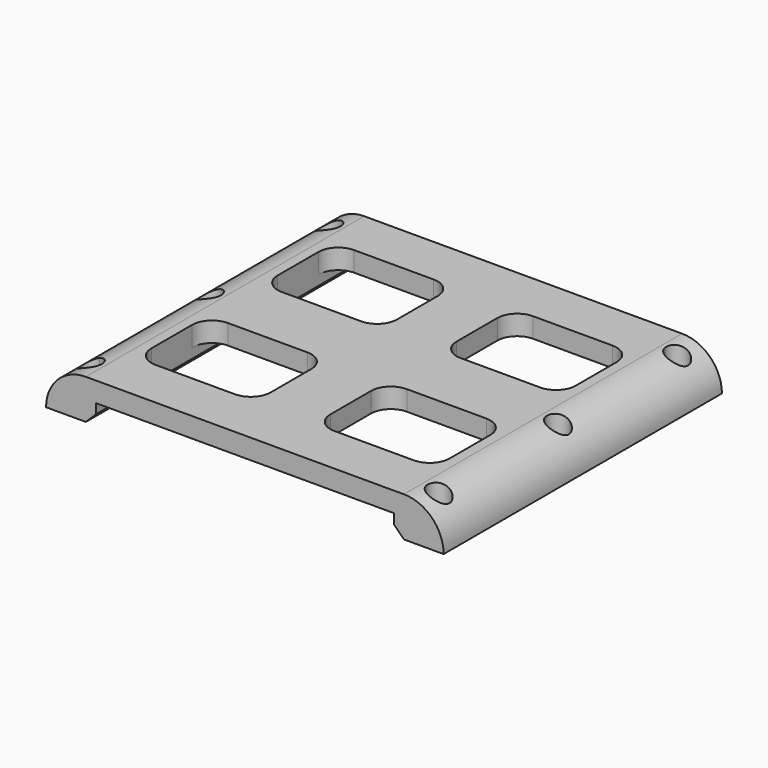
from build123d import *

# Parameters (mm, degrees)
F1_DEPTH    = 44.45
F2_R        = 5.07999
F3_R        = 1.397
F4_DEPTH    = 25.4
F5_W        = 15.24
F5_H        = 11.5777312835
F6_DEPTH    = 25.4
F7_R        = 2.54
F8_T1_DEPTH = 50.9820747894


# Not quite as in the source:
# - a fillet or chamfer that OpenCascade refuses, or shapes differently, is made with other operations: its cross-section is extruded or revolved along the edge and cut away or added
# - a fillet or chamfer is up to 0.001 mm smaller than in the source, because OpenCascade refuses the exact size


with BuildPart() as f1:
    # F0 (on Front) → F1 (new body)
    with BuildSketch(Plane.XZ):
        Polygon((0, 1.27), (-25.4, 1.27), (-25.4, -1.27), (-25.4, -3.81), (-19.05, -3.81), (-19.05, -1.27), (19.05, -1.27), (19.05, -3.81), (25.4, -3.81), (25.4, -1.27), (25.4, 1.27), align=None)
    extrude(amount=F1_DEPTH)

    # F2 (radius 5.08 in the source; OpenCascade refuses exactly that, so slightly less here)
    f2_edges = [f1.edges().sort_by_distance(p)[0] for p in [
        (-25.4, -22.225, 1.27),
        (25.4, -22.225, 1.27),
    ]]
    fillet(f2_edges, radius=F2_R)

    # F3 (on face) → F4 (cut)
    with BuildSketch(Plane(origin=(0, 0, -3.81), x_dir=(1, 0, 0), z_dir=(0, 0, -1))):
        with BuildLine():
            ThreePointArc((-22.225, 23.622), (-23.2128281733, 21.2371718267), (-20.828, 22.225))
            Line((-20.828, 22.225), (-22.225, 22.225))
            Line((-22.225, 22.225), (-22.225, 23.622))
        make_face()
        with BuildLine():
            Line((-22.225, 22.225), (-20.828, 22.225))
            ThreePointArc((-20.828, 22.225), (-21.2371718267, 23.2128281733), (-22.225, 23.622))
            Line((-22.225, 23.622), (-22.225, 22.225))
        make_face()
        with BuildLine():
            ThreePointArc((-22.225, 42.672), (-23.622, 41.275), (-22.225, 39.878))
            Line((-22.225, 39.878), (-22.225, 41.275))
            Line((-22.225, 41.275), (-22.225, 42.672))
        make_face()
        with BuildLine():
            Line((-22.225, 41.275), (-22.225, 39.878))
            ThreePointArc((-22.225, 39.878), (-21.2371718267, 40.2871718267), (-20.828, 41.275))
            ThreePointArc((-20.828, 41.275), (-21.2371718267, 42.2628281733), (-22.225, 42.672))
            Line((-22.225, 42.672), (-22.225, 41.275))
        make_face()
        with Locations((-22.225, 3.175)):
            Circle(F3_R)
        with Locations((22.225, 41.275)):
            Circle(F3_R)
        with Locations((22.225, 3.175)):
            Circle(F3_R)
        with Locations((22.225, 22.225)):
            Circle(F3_R)
    extrude(amount=-F4_DEPTH, mode=Mode.SUBTRACT)

    # F5 (on face) → F6 (cut)
    with BuildSketch(Plane.XY.offset(1.27)):
        with Locations((11.43, -12.1388656418)):
            Rectangle(F5_W, F5_H)
        with Locations((-11.43, -12.1388656418)):
            Rectangle(F5_W, F5_H)
        with Locations((11.43, -32.3111343582)):
            Rectangle(F5_W, F5_H)
        with Locations((-11.43, -32.3111343582)):
            Rectangle(F5_W, F5_H)
    extrude(amount=-F6_DEPTH, mode=Mode.SUBTRACT)

    # F7
    f7_edges = [f1.edges().sort_by_distance(p)[0] for p in [
        (-19.05, -6.35, 0),
        (-3.81, -17.927731, 0),
        (-3.81, -6.35, 0),
        (-19.05, -17.927731, 0),
        (-19.05, -38.1, 0),
        (3.81, -38.1, 0),
        (3.81, -17.927731, 0),
        (3.81, -6.35, 0),
        (-19.05, -26.522269, 0),
        (3.81, -26.522269, 0),
        (19.05, -26.522269, 0),
        (-3.81, -26.522269, 0),
        (19.05, -6.35, 0),
        (19.05, -17.927731, 0),
        (19.05, -38.1, 0),
        (-3.81, -38.1, 0),
    ]]
    fillet(f7_edges, radius=F7_R)

    # F8: chamfer of 1.27 on 14 edges, made by hand

    # F8_s2 → F8_t1 (cut)
    with BuildSketch(Plane.XZ.offset(-3.2660373947)):
        Polygon((19.05, -2.54), (20.32, -3.81), (19.05, -3.81), align=None)
        Polygon((-19.05, -2.54), (-20.32, -3.81), (-19.05, -3.81), align=None)
    extrude(amount=F8_T1_DEPTH, mode=Mode.SUBTRACT)


solid = f1.part
